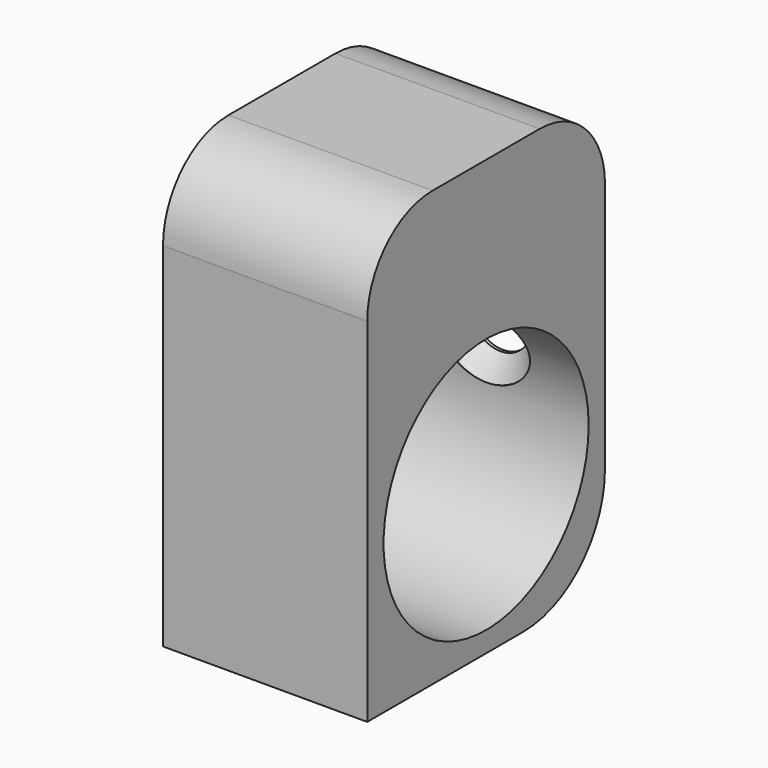
from build123d import *

# Parameters (mm, degrees)
F0_R     = 12.55
F0_R_2   = 2.75
F0_R_3   = 4
F1_DEPTH = 10
F2_R     = 10
F3_R     = 2.9
F4_DEPTH = 14.551
F3_R_2   = 5
F5_DEPTH = 12.5


with BuildPart() as f1:
    # F0 (on Right) → F1 (new body, symmetric)
    with BuildSketch(Plane.YZ):
        with BuildLine():
            ThreePointArc((14.55, 20), (12.2068542495, 25.6568542495), (6.55, 28))
            Line((6.55, 28), (-6.55, 28))
            ThreePointArc((-6.55, 28), (-12.2068542495, 25.6568542495), (-14.55, 20))
            Line((-14.55, 20), (-14.55, -14.55))
            Line((-14.55, -14.55), (14.55, -14.55))
            Line((14.55, -14.55), (14.55, 20))
        make_face()
        Circle(F0_R, mode=Mode.SUBTRACT)
        with Locations((-6.8404028665, 18.7938524157)):
            Circle(F0_R_2, mode=Mode.SUBTRACT)
        with Locations((6.8404028665, 18.7938524157)):
            Circle(F0_R_3, mode=Mode.SUBTRACT)
        with Locations((6.8404028665, 18.7938524157)):
            Circle(F0_R_3)
        with Locations((-6.8404028665, 18.7938524157)):
            Circle(F0_R_2)
    extrude(amount=F1_DEPTH, both=True)

    # F2
    f2_edges = [f1.edges().sort_by_distance(p)[0] for p in [
        (0, 14.55, -14.55),
    ]]
    fillet(f2_edges, radius=F2_R)

    # F3 (on Front) → F4 (cut, through all)
    with BuildSketch(Plane.XZ):
        with Locations((0, 5.45)):
            Circle(F3_R)
    extrude(amount=-F4_DEPTH, mode=Mode.SUBTRACT)

    # F3 (on Front) → F5 (cut)
    with BuildSketch(Plane.XZ):
        with Locations((0, 5.45)):
            Circle(F3_R_2)
        with Locations((0, 5.45)):
            Circle(F3_R, mode=Mode.SUBTRACT)
    extrude(amount=-F5_DEPTH, mode=Mode.SUBTRACT)

    # F6 (on Right) → F7 (revolve, cut)
    with BuildSketch(Plane.YZ):
        Polygon((14.55, 5.45), (14.55, 8.45), (14.25, 8.45), (12.55, 10.45), (11.55, 10.45), (11.55, 5.45), align=None)
    revolve(axis=Axis((0, 7.275, 5.45), (0, 1, 0)), mode=Mode.SUBTRACT)


solid = f1.part
